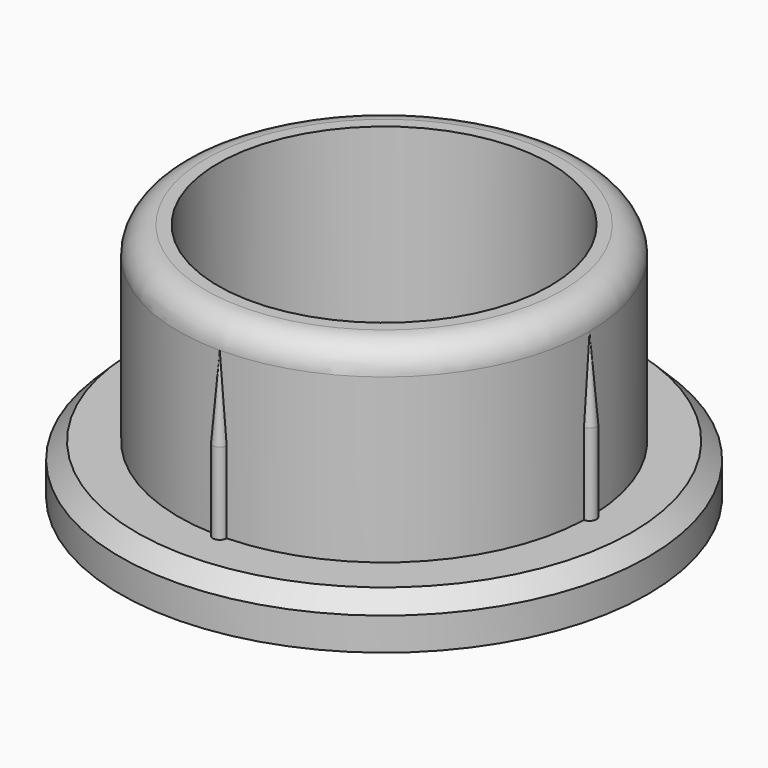
from build123d import *

# Parameters (mm, degrees)
F0_R         = 48.5
F0_R_2       = 30.5
F1_DEPTH     = 9
F2_R         = 37.75
F2_R_2       = 30.5
F3_DEPTH     = 35
F4_R         = 5
F5_R         = 1.25
F5_R_2       = 1.255
F6_DEPTH     = 30
F7_T4_ANGLE  = 359.64
F7_S5_R      = 37.75
F7_T6_DEPTH  = 9
F7_T10_ANGLE = 359.64
F7_S11_R     = 37.75
F7_T12_DEPTH = 9
F7_T16_ANGLE = 359.64
F7_S17_R     = 37.75
F7_T18_DEPTH = 9
F7_T22_ANGLE = 359.64
F7_S23_R     = 37.75
F7_T24_DEPTH = 9
F8_SIZE      = 2
F9_SIZE      = 3


# Not quite as in the source:
# - a fillet or chamfer that OpenCascade refuses, or shapes differently, is made with other operations: its cross-section is extruded or revolved along the edge and cut away or added


with BuildPart() as f1:
    # F0 (on Top) → F1 (new body)
    with BuildSketch(Plane.XY):
        Circle(F0_R)
        Circle(F0_R_2, mode=Mode.SUBTRACT)
    extrude(amount=F1_DEPTH)

    # F2 (on face) → F3 (join)
    with BuildSketch(Plane.XY.offset(9)):
        Circle(F2_R)
        Circle(F2_R_2, mode=Mode.SUBTRACT)
    extrude(amount=F3_DEPTH)

    # F4
    f4_edges = [f1.edges().sort_by_distance(p)[0] for p in [
        (-37.75, 0, 44),
    ]]
    fillet(f4_edges, radius=F4_R)

    # F5 (on face) → F6 (join)
    with BuildSketch(Plane.XY.offset(9)):
        with Locations((0, 37.75)):
            Circle(F5_R)
        with Locations((-37.75, 0)):
            Circle(F5_R_2)
        with Locations((0, -37.75)):
            Circle(F5_R_2)
        with Locations((37.75, 0)):
            Circle(F5_R_2)
    extrude(amount=F6_DEPTH)

    # F7: chamfer of 1.249 x 15 on 4 edges, made by hand


with BuildPart() as f7_tool2:
    # F7_s3 → F7_t4 (revolve)
    with BuildSketch(Plane(origin=(-0.0003725763, 0.1185943423, 0), x_dir=(0, 0, 1), z_dir=(0.0031415875, -0.9999950652, 0))):
        Polygon((24, 36.4948137114), (39, 37.7438137114), (39, 36.4948137114), align=None)
    revolve(axis=Axis((-37.75, 0, 39), (0, 0, 1)), revolution_arc=F7_T4_ANGLE)

    # F7_s5 → F7_t6 (cut, symmetric)
    with BuildSketch(Plane.XY.offset(31.5)):
        Circle(F7_S5_R)
    extrude(amount=F7_T6_DEPTH, both=True, mode=Mode.SUBTRACT)


with BuildPart() as f1_1:
    add(f1.part)

    # F7_t1: cut F7_tool2
    add(f7_tool2.part, mode=Mode.SUBTRACT)


with BuildPart() as f7_tool8:
    # F7_s9 → F7_t10 (revolve)
    with BuildSketch(Plane(origin=(0.1185943423, 0.0003725763, 0), x_dir=(0, 0, 1), z_dir=(-0.9999950652, -0.0031415875, 0))):
        Polygon((24, 36.4998137114), (39, 37.7488137114), (39, 36.4998137114), align=None)
    revolve(axis=Axis((0, 37.75, 39), (0, 0, 1)), revolution_arc=F7_T10_ANGLE)

    # F7_s11 → F7_t12 (cut, symmetric)
    with BuildSketch(Plane.XY.offset(31.5)):
        Circle(F7_S11_R)
    extrude(amount=F7_T12_DEPTH, both=True, mode=Mode.SUBTRACT)


with BuildPart() as f1_2:
    add(f1_1.part)

    # F7_t7: cut F7_tool8
    add(f7_tool8.part, mode=Mode.SUBTRACT)


with BuildPart() as f7_tool14:
    # F7_s15 → F7_t16 (revolve)
    with BuildSketch(Plane(origin=(-0.1185943423, -0.0003725763, 0), x_dir=(0, 0, 1), z_dir=(0.9999950652, 0.0031415875, 0))):
        Polygon((24, 36.4948137114), (39, 37.7438137114), (39, 36.4948137114), align=None)
    revolve(axis=Axis((0, -37.75, 39), (0, 0, 1)), revolution_arc=F7_T16_ANGLE)

    # F7_s17 → F7_t18 (cut, symmetric)
    with BuildSketch(Plane.XY.offset(31.5)):
        Circle(F7_S17_R)
    extrude(amount=F7_T18_DEPTH, both=True, mode=Mode.SUBTRACT)


with BuildPart() as f1_3:
    add(f1_2.part)

    # F7_t13: cut F7_tool14
    add(f7_tool14.part, mode=Mode.SUBTRACT)


with BuildPart() as f7_tool20:
    # F7_s21 → F7_t22 (revolve)
    with BuildSketch(Plane(origin=(0.0003725763, -0.1185943423, 0), x_dir=(0, 0, 1), z_dir=(-0.0031415875, 0.9999950652, 0))):
        Polygon((24, 36.4948137114), (39, 37.7438137114), (39, 36.4948137114), align=None)
    revolve(axis=Axis((37.75, 0, 39), (0, 0, 1)), revolution_arc=F7_T22_ANGLE)

    # F7_s23 → F7_t24 (cut, symmetric)
    with BuildSketch(Plane.XY.offset(31.5)):
        Circle(F7_S23_R)
    extrude(amount=F7_T24_DEPTH, both=True, mode=Mode.SUBTRACT)


with BuildPart() as f1_4:
    add(f1_3.part)

    # F7_t19: cut F7_tool20
    add(f7_tool20.part, mode=Mode.SUBTRACT)

    # F8
    f8_edges = [f1_4.edges().sort_by_distance(p)[0] for p in [
        (-30.5, 0, 0),
    ]]
    chamfer(f8_edges, length=F8_SIZE)

    # F9
    f9_edges = [f1_4.edges().sort_by_distance(p)[0] for p in [
        (-48.5, 0, 9),
    ]]
    chamfer(f9_edges, length=F9_SIZE)


solid = f1_4.part
